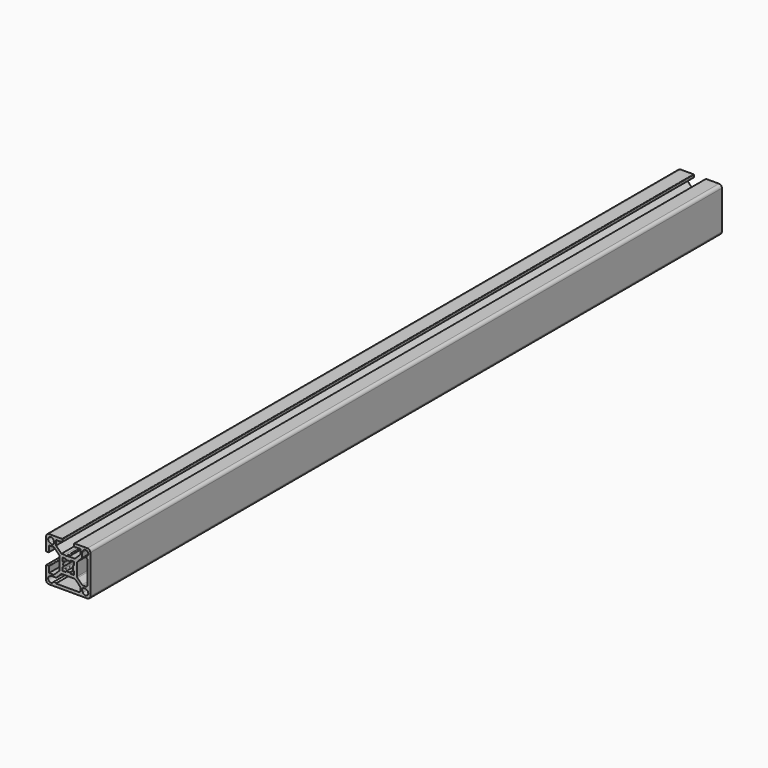
from build123d import *

# Parameters (mm, degrees)
F2_DEPTH = 267.5


# Not quite as in the source:
# - ends of sketch curves that miss each other by under 0.0002 mm in the source are joined


with BuildPart() as f2:
    # F1 (on Front) → F2 (new body, symmetric)
    with BuildSketch(Plane.XZ):
        with BuildLine():
            Line((-8.250056, 12.999986), (-4.300056, 12.999986))
            ThreePointArc((-4.300056, 12.999986), (-4.0879239656, 13.0878539656), (-4.000056, 13.299986))
            Line((-4.000056, 13.299986), (-4.000056, 14.699986))
            ThreePointArc((-4.000056, 14.699986), (-4.0879239656, 14.9121180344), (-4.300056, 14.999986))
            Line((-4.300056, 14.999986), (-13.000056, 14.999986))
            ThreePointArc((-13.000056, 14.999986), (-14.4142695624, 14.4141995624), (-15.000056, 12.999986))
            Line((-15.000056, 12.999986), (-15.000056, 4.299986))
            ThreePointArc((-15.000056, 4.299986), (-14.9121880344, 4.0878539656), (-14.700056, 3.999986))
            Line((-14.700056, 3.999986), (-13.300056, 3.999986))
            ThreePointArc((-13.300056, 3.999986), (-13.0879239656, 4.0878539656), (-13.000056, 4.299986))
            Line((-13.000056, 4.299986), (-13.000056, 8.249986))
            Line((-13.000056, 8.249986), (-9.66427, 8.249986))
            Line((-9.66427, 8.249986), (-6.000056, 4.585772))
            Line((-6.000056, 4.585772), (-6.000056, 0.653576))
            ThreePointArc((-6.000056, 0.653576), (-5.9830189324, 0.5241665494), (-5.9330687764, 0.4035761291))
            Line((-5.9330687764, 0.4035761291), (-5.700056, -1.4e-05))
            Line((-5.700056, -1.4e-05), (-5.933069, -0.403604))
            ThreePointArc((-5.933069, -0.403604), (-6.000056, -0.653604), (-5.9330687764, -0.9036038709))
            Line((-5.9330687764, -0.9036038709), (-5.751033, -1.2189))
            Line((-5.751033, -1.2189), (-6.000056, -2.500014))
            Line((-6.000056, -2.500014), (-6.000056, -4.5858))
            Line((-6.000056, -4.5858), (-9.66427, -8.250014))
            Line((-9.66427, -8.250014), (-13.000056, -8.250014))
            Line((-13.000056, -8.250014), (-13.000056, -4.300014))
            ThreePointArc((-13.000056, -4.300014), (-13.0879239656, -4.0878819656), (-13.300056, -4.000014))
            Line((-13.300056, -4.000014), (-14.700056, -4.000014))
            ThreePointArc((-14.700056, -4.000014), (-14.9121880344, -4.0878819656), (-15.000056, -4.300014))
            Line((-15.000056, -4.300014), (-15.000056, -13.000014))
            ThreePointArc((-15.000056, -13.000014), (-14.4142695624, -14.4142275624), (-13.000056, -15.000014))
            Line((-13.000056, -15.000014), (12.999944, -15.000014))
            ThreePointArc((12.999944, -15.000014), (14.4141575624, -14.4142275624), (14.999944, -13.000014))
            Line((14.999944, -13.000014), (14.999944, 12.999986))
            ThreePointArc((14.999944, 12.999986), (14.4141575624, 14.4141995624), (12.999944, 14.999986))
            Line((12.999944, 14.999986), (4.299944, 14.999986))
            ThreePointArc((4.299944, 14.999986), (4.0878119656, 14.9121180344), (3.999944, 14.699986))
            Line((3.999944, 14.699986), (3.999944, 13.299986))
            ThreePointArc((3.999944, 13.299986), (4.0878119656, 13.0878539656), (4.299944, 12.999986))
            Line((4.299944, 12.999986), (8.249944, 12.999986))
            Line((8.249944, 12.999986), (8.249944, 9.6642))
            Line((8.249944, 9.6642), (4.58573, 5.999986))
            Line((4.58573, 5.999986), (0.653534, 5.999986))
            ThreePointArc((0.653534, 5.999986), (0.5241245494, 5.9829489324), (0.4035341291, 5.9329987764))
            Line((0.4035341291, 5.9329987764), (-5.6e-05, 5.699986))
            Line((-5.6e-05, 5.699986), (-0.403646, 5.932999))
            ThreePointArc((-0.403646, 5.932999), (-0.653646, 5.999986), (-0.9036458709, 5.9329987764))
            Line((-0.9036458709, 5.9329987764), (-1.218942, 5.750963))
            Line((-1.218942, 5.750963), (-2.500056, 5.999986))
            Line((-2.500056, 5.999986), (-4.585842, 5.999986))
            Line((-4.585842, 5.999986), (-8.250056, 9.6642))
            Line((-8.250056, 9.6642), (-8.250056, 12.999986))
        make_face()
        with BuildLine():
            ThreePointArc((-8.189375, -13.000014), (-8.339375082, -12.9598215738), (-8.4491827159, -12.8500138359))
            ThreePointArc((-8.4491827159, -12.8500138359), (-9.2743948384, -12.3508472042), (-10.1375690315, -12.7810479782))
            ThreePointArc((-10.1375690315, -12.7810479782), (-13.2041723505, -12.8608903949), (-12.3498940253, -9.9145979306))
            Line((-12.3498940253, -9.9145979306), (-11.07346, -9.450014))
            Line((-11.07346, -9.450014), (-8.450056, -9.450014))
            ThreePointArc((-8.450056, -9.450014), (-8.0673725676, -9.3738935325), (-7.7429492188, -9.1571207812))
            Line((-7.7429492188, -9.1571207812), (-4.878736, -6.292907))
            ThreePointArc((-4.878736, -6.292907), (-4.5543124324, -6.0761344675), (-4.171629, -6.000014))
            Line((-4.171629, -6.000014), (4.171517, -6.000014))
            ThreePointArc((4.171517, -6.000014), (4.5542004324, -6.0761344675), (4.8786237812, -6.2929072188))
            Line((4.8786237812, -6.2929072188), (7.957051, -9.371334))
            ThreePointArc((7.957051, -9.371334), (8.1738235325, -9.6957575676), (8.249944, -10.078441))
            Line((8.249944, -10.078441), (8.249944, -12.000014))
            ThreePointArc((8.249944, -12.000014), (7.9570507812, -12.7071207812), (7.249944, -13.000014))
            Line((7.249944, -13.000014), (-8.189375, -13.000014))
        make_face(mode=Mode.SUBTRACT)
        with BuildLine():
            ThreePointArc((9.5477956661, -11.3422641215), (9.8734155063, -9.8734855063), (11.3421941215, -9.5478656661))
            Line((11.3421941215, -9.5478656661), (12.349782, -9.914598))
            ThreePointArc((12.349782, -9.914598), (13.0434468843, -13.0435168843), (9.9145279306, -12.3498520253))
            Line((9.9145279306, -12.3498520253), (9.5477956661, -11.3422641215))
        make_face(mode=Mode.SUBTRACT)
        with BuildLine():
            ThreePointArc((-9.5479076661, 11.3422361215), (-9.8735275063, 9.8734575063), (-11.3423061215, 9.5478376661))
            Line((-11.3423061215, 9.5478376661), (-12.349894, 9.91457))
            ThreePointArc((-12.349894, 9.91457), (-13.0435588843, 13.0434888843), (-9.9146399306, 12.3498240253))
            Line((-9.9146399306, 12.3498240253), (-9.5479076661, 11.3422361215))
        make_face(mode=Mode.SUBTRACT)
        with BuildLine():
            ThreePointArc((3.2531309855, 0.9883049956), (3.399944, -1.4e-05), (3.2531309855, -0.9883329956))
            ThreePointArc((3.2531309855, -0.9883329956), (3.2974111593, -1.3177976431), (3.5754529349, -1.5000144258))
            ThreePointArc((3.5754529349, -1.5000144258), (3.8792555231, -1.6685151025), (3.999944, -1.99428))
            Line((3.999944, -1.99428), (3.999944, -3.500014))
            ThreePointArc((3.999944, -3.500014), (3.8534973906, -3.8535673906), (3.499944, -4.000014))
            Line((3.499944, -4.000014), (1.99421, -4.000014))
            ThreePointArc((1.99421, -4.000014), (1.6684451025, -3.8793255231), (1.4999444822, -3.5755229263))
            ThreePointArc((1.4999444822, -3.5755229263), (1.3177276431, -3.2974811593), (0.9882590481, -3.2532021585))
            ThreePointArc((0.9882590481, -3.2532021585), (-5.6e-05, -3.400014), (-0.9883749956, -3.2532009855))
            ThreePointArc((-0.9883749956, -3.2532009855), (-1.3178396431, -3.2974811593), (-1.5000564258, -3.5755229349))
            ThreePointArc((-1.5000564258, -3.5755229349), (-1.6685571025, -3.8793255231), (-1.994322, -4.000014))
            Line((-1.994322, -4.000014), (-3.500056, -4.000014))
            ThreePointArc((-3.500056, -4.000014), (-3.8536093906, -3.8535673906), (-4.000056, -3.500014))
            Line((-4.000056, -3.500014), (-4.000056, -1.99428))
            ThreePointArc((-4.000056, -1.99428), (-3.8793675231, -1.6685151025), (-3.5755649263, -1.5000144822))
            ThreePointArc((-3.5755649263, -1.5000144822), (-3.2975231593, -1.3177976431), (-3.2532441585, -0.9883290481))
            ThreePointArc((-3.2532441585, -0.9883290481), (-3.400056, -1.4e-05), (-3.2532429855, 0.9883049956))
            ThreePointArc((-3.2532429855, 0.9883049956), (-3.2975231593, 1.3177696431), (-3.5755649349, 1.4999864258))
            ThreePointArc((-3.5755649349, 1.4999864258), (-3.8793675231, 1.6684871025), (-4.000056, 1.994252))
            Line((-4.000056, 1.994252), (-4.000056, 3.499986))
            ThreePointArc((-4.000056, 3.499986), (-3.8536093906, 3.8535393906), (-3.500056, 3.999986))
            Line((-3.500056, 3.999986), (-1.994322, 3.999986))
            ThreePointArc((-1.994322, 3.999986), (-1.6685571025, 3.8792975231), (-1.5000564822, 3.5754949263))
            ThreePointArc((-1.5000564822, 3.5754949263), (-1.3178396431, 3.2974531593), (-0.9883710481, 3.2531741585))
            ThreePointArc((-0.9883710481, 3.2531741585), (-5.6e-05, 3.399986), (0.9882629956, 3.2531729855))
            ThreePointArc((0.9882629956, 3.2531729855), (1.3177276431, 3.2974531593), (1.4999444258, 3.5754949349))
            ThreePointArc((1.4999444258, 3.5754949349), (1.6684451025, 3.8792975231), (1.99421, 3.999986))
            Line((1.99421, 3.999986), (3.499944, 3.999986))
            ThreePointArc((3.499944, 3.999986), (3.8534973906, 3.8535393906), (3.999944, 3.499986))
            Line((3.999944, 3.499986), (3.999944, 1.994252))
            ThreePointArc((3.999944, 1.994252), (3.8792555231, 1.6684871025), (3.5754529263, 1.4999864822))
            ThreePointArc((3.5754529263, 1.4999864822), (3.2974111593, 1.3177696431), (3.2531309855, 0.9883049956))
        make_face(mode=Mode.SUBTRACT)
        with BuildLine():
            ThreePointArc((6.2928372188, -4.8786937812), (6.0760644675, -4.5542704324), (5.999944, -4.171587))
            Line((5.999944, -4.171587), (5.999944, 4.171559))
            ThreePointArc((5.999944, 4.171559), (6.0760644675, 4.5542424324), (6.2928372188, 4.8786657812))
            Line((6.2928372188, 4.8786657812), (9.157051, 7.742879))
            ThreePointArc((9.157051, 7.742879), (9.3738235325, 8.0673025676), (9.449944, 8.449986))
            Line((9.449944, 8.449986), (9.449944, 11.07339))
            Line((9.449944, 11.07339), (9.914528, 12.349824))
            ThreePointArc((9.914528, 12.349824), (12.8608203949, 13.2041023505), (12.7809779799, 10.1374990291))
            ThreePointArc((12.7809779799, 10.1374990291), (12.3507772042, 9.2743248384), (12.8499438252, 8.4491126972))
            ThreePointArc((12.8499438252, 8.4491126972), (12.9597515738, 8.339305082), (12.999944, 8.189305))
            Line((12.999944, 8.189305), (12.999944, -7.250014))
            ThreePointArc((12.999944, -7.250014), (12.7070507812, -7.9571207812), (11.999944, -8.250014))
            Line((11.999944, -8.250014), (10.078371, -8.250014))
            ThreePointArc((10.078371, -8.250014), (9.6956875676, -8.1738935325), (9.3712642188, -7.9571207812))
            Line((9.3712642188, -7.9571207812), (6.2928372188, -4.8786937812))
        make_face(mode=Mode.SUBTRACT)
    extrude(amount=F2_DEPTH, both=True)


solid = f2.part
